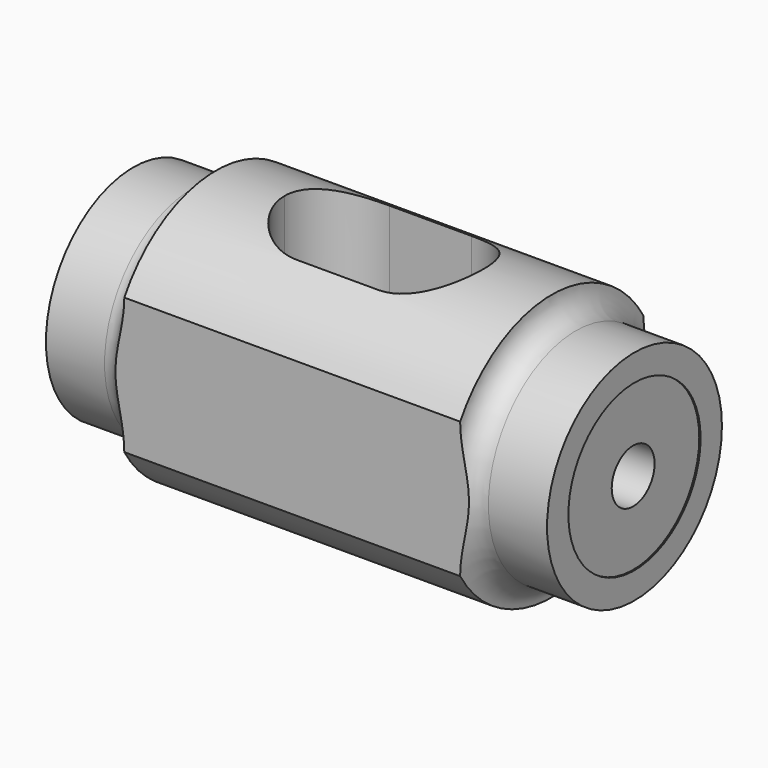
from build123d import *

# Parameters (mm, degrees)
F2_W     = 38.091527
F2_H     = 5.860234
F3_DEPTH = 12.7
F4_R     = 7.874
F5_DEPTH = 0.127
F7_D     = 5.1054
F7_DEPTH = 12.7
F7_TIP   = 1.533817
F8_R     = 6.35
F9_DEPTH = 12.7


with BuildPart() as f1:
    # F0 (on Top) → F1 (revolve)
    with BuildSketch(Plane.XY):
        with BuildLine():
            Line((16.002, 12.7), (-16.002, 12.7))
            ThreePointArc((-16.002, 12.7), (-16.671554, 11.083554), (-18.288, 10.414))
            Line((-18.288, 10.414), (-23.876, 10.414))
            Line((-23.876, 10.414), (-23.876, 0))
            Line((-23.876, 0), (23.876, 0))
            Line((23.876, 0), (23.876, 10.414))
            Line((23.876, 10.414), (18.288, 10.414))
            ThreePointArc((18.288, 10.414), (16.671554, 11.083554), (16.002, 12.7))
        make_face()
    revolve(axis=Axis((0.053952, 0, 0), (1, 0, 0)))

    # F2 (on Top) → F3 (cut, symmetric)
    with BuildSketch(Plane.XY):
        with Locations((0.198507, 13.852117)):
            Rectangle(F2_W, F2_H)
        with Locations((0.198507, -13.852117)):
            Rectangle(F2_W, F2_H)
        with BuildLine():
            ThreePointArc((9.4615, 0), (7.832252, 3.933352), (3.8989, 5.5626))
            Line((3.8989, 5.5626), (-3.8989, 5.5626))
            ThreePointArc((-3.8989, 5.5626), (-7.832252, 3.933352), (-9.4615, 0))
            ThreePointArc((-9.4615, 0), (-7.832252, -3.933352), (-3.8989, -5.5626))
            Line((-3.8989, -5.5626), (3.8989, -5.5626))
            ThreePointArc((3.8989, -5.5626), (7.832252, -3.933352), (9.4615, 0))
        make_face()
    extrude(amount=F3_DEPTH, both=True, mode=Mode.SUBTRACT)

    # F4 (on face) → F5 (cut)
    with BuildSketch(Plane.YZ.offset(23.876)):
        Circle(F4_R)
    extrude(amount=-F5_DEPTH, mode=Mode.SUBTRACT)

    # F7
    with Locations(Plane.YZ.offset(23.749)):
        with Locations((0, 0)):
            Hole(F7_D / 2, depth=F7_DEPTH)
            with Locations((0, 0, -(F7_DEPTH + F7_TIP / 2))):  # 118° drill point
                Cone(0, F7_D / 2, F7_TIP, mode=Mode.SUBTRACT)

    # F8 (on face) → F9 (cut)
    with BuildSketch(Plane(origin=(-23.876, 0, 0), x_dir=(0, -1, 0), z_dir=(-1, 0, 0))):
        Circle(F8_R)
    extrude(amount=-F9_DEPTH, mode=Mode.SUBTRACT)


solid = f1.part
